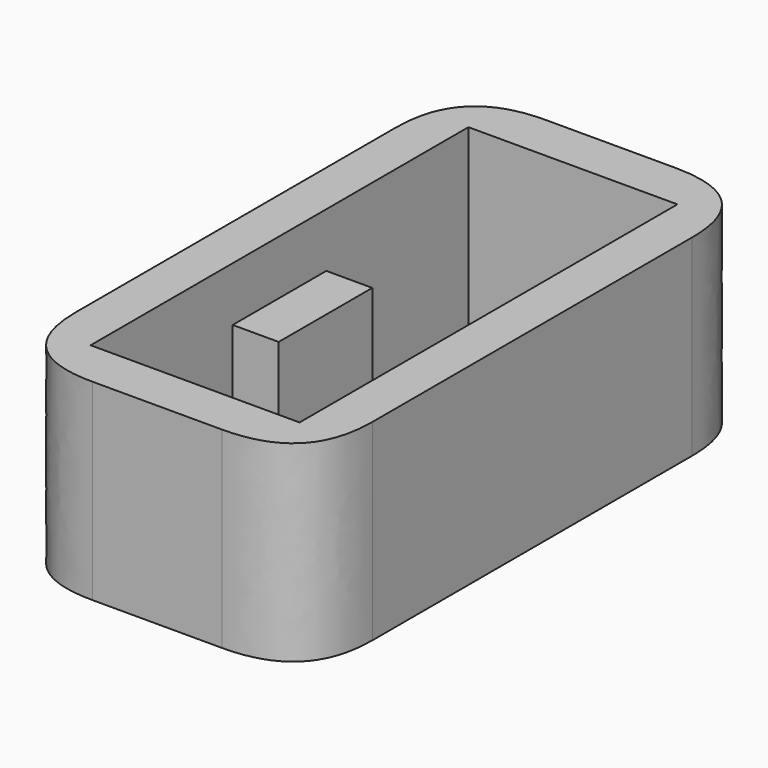
from build123d import *

# Parameters (mm, degrees)
F0_W        = 9.017
F0_H        = 17.2212
F0_W_2      = 6.35
F0_H_2      = 14.351
F1_DEPTH    = 5.842
F2_T1_DEPTH = 18.542
F3_W        = 3.556
F3_H        = 2.54
F4_DEPTH    = 1.397


# Not quite as in the source:
# - a fillet or chamfer that OpenCascade refuses, or shapes differently, is made with other operations: its cross-section is extruded or revolved along the edge and cut away or added


with BuildPart() as f1:
    # F0 (on Top) → F1 (new body)
    with BuildSketch(Plane.XY):
        Rectangle(F0_W, F0_H)
        Rectangle(F0_W_2, F0_H_2, mode=Mode.SUBTRACT)
    extrude(amount=F1_DEPTH)

    # F2: fillet of radius 2.54 on 4 edges, made by hand

    # F2_s2 → F2_t1 (cut)
    with BuildSketch(Plane.XY.offset(-6.35)):
        with BuildLine():
            add(Edge.make_bspline(
                [(-1.9685, 8.6106), (-4.5085, 8.6106), (-4.5085, 6.0706)],
                knots=[0, 0, 0, 1, 1, 1], degree=2, weights=[1, 1, 1]))
            Line((-4.5085, 6.0706), (-4.5085, 8.6106))
            Line((-4.5085, 8.6106), (-1.9685, 8.6106))
        make_face()
        with BuildLine():
            add(Edge.make_bspline(
                [(-1.9685, -8.6106), (-4.5085, -8.6106), (-4.5085, -6.0706)],
                knots=[0, 0, 0, 1, 1, 1], degree=2, weights=[1, 1, 1]))
            Line((-4.5085, -6.0706), (-4.5085, -8.6106))
            Line((-4.5085, -8.6106), (-1.9685, -8.6106))
        make_face()
        with BuildLine():
            add(Edge.make_bspline(
                [(1.9685, -8.6106), (4.5085, -8.6106), (4.5085, -6.0706)],
                knots=[0, 0, 0, 1, 1, 1], degree=2, weights=[1, 1, 1]))
            Line((4.5085, -6.0706), (4.5085, -8.6106))
            Line((4.5085, -8.6106), (1.9685, -8.6106))
        make_face()
        with BuildLine():
            add(Edge.make_bspline(
                [(4.5085, 6.0706), (4.5085, 8.6106), (1.9685, 8.6106)],
                knots=[0, 0, 0, 1, 1, 1], degree=2, weights=[1, 1, 1]))
            Line((1.9685, 8.6106), (4.5085, 8.6106))
            Line((4.5085, 8.6106), (4.5085, 6.0706))
        make_face()
    extrude(amount=F2_T1_DEPTH, mode=Mode.SUBTRACT)


with BuildPart() as f4:
    # F3 (on face) → F4 (new body)
    with BuildSketch(Plane.YZ.offset(-3.175)):
        with Locations((0, 2.921)):
            Rectangle(F3_W, F3_H)
    extrude(amount=F4_DEPTH)


solid = Compound([f1.part, f4.part])
